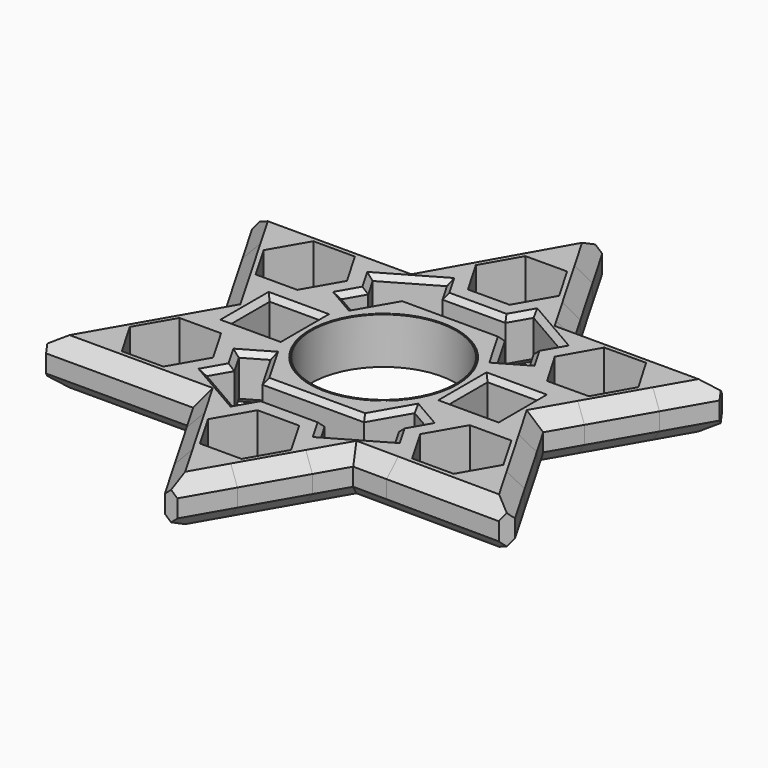
from build123d import *

# Parameters (mm, degrees)
F0_W     = 2.54
F0_H     = 8.7372876405
F0_H_2   = 8.9837514889
F1_DEPTH = 6.9977
F0_R     = 11.0653677003
F0_R_2   = 10.9474
F2_R     = 11.176
F3_DEPTH = 6.9977
F4_SIZE  = 2.159
F5_W     = 7.62
F5_H     = 7.62
F6_DEPTH = 25.4
F7_SIZE  = 0.762


with BuildPart() as f1:
    # F0 (on Top) → F1 (new body)
    with BuildSketch(Plane.XY):
        Polygon((12.5002051005, 12.7937514889), (14.280010725, 9.7110377198), (15.550010725, 7.5113331942), (17.2662315727, 4.5387514889), (20.7270452561, 4.5387514889), (23.2670452561, 4.5387514889), (26.798284517, 4.5387514889), (31.5643109892, 12.7937514889), (26.798284517, 21.0487514889), (17.2662315727, 21.0487514889), (15.5094151394, 18.0058561669), (14.1988195539, 15.7358380246), align=None)
        Polygon((25.2207365934, 7.3534421339), (18.9150512132, 7.3122933889), (15.7265726647, 12.7526027439), (18.8437794963, 18.2340608439), (25.1494648765, 18.2752095889), (28.3379434251, 12.8349002339), align=None, mode=Mode.SUBTRACT)
        Polygon((35.3419193782, -19.304), (31.5290982004, -12.7), (26.7630717283, -20.955), (17.231018784, -20.955), (34.3130483735, -21.0860568545), align=None)
        Polygon((4.7660264722, -33.655), (-4.7660264722, -33.655), (-0.9532052944, -40.259), (0.9532052944, -40.259), align=None)
        Polygon((-14.2130055479, -9.6723522628), (-15.4830055479, -7.4726477372), (-17.231018784, -4.445), (-20.7270452561, -4.445), (-23.2670452561, -4.445), (-26.7630717283, -4.445), (-31.5290982004, -12.7), (-26.7630717283, -20.955), (-17.231018784, -20.955), (-15.4830055479, -17.9273522628), (-14.2130055479, -15.7276477372), (-12.4649923118, -12.7), align=None)
        Polygon((-25.1531495269, -7.2408455632), (-18.847330966, -7.2371563061), (-15.6912266952, -12.6963107429), (-18.8409409854, -18.1591544368), (-25.1467595462, -18.1628436939), (-28.302863817, -12.7036892571), align=None, mode=Mode.SUBTRACT)
        with Locations((-21.9970452561, -0.0763561798)):
            Rectangle(F0_W, F0_H)
        Polygon((-35.2537508563, 19.1512876405), (-31.4409296786, 12.5472876405), (-29.0579164425, 16.6747876405), (-34.7771482091, 19.9767876405), align=None)
        Polygon((-29.0579164425, 16.6747876405), (-26.6749032064, 20.8022876405), (-34.3005455619, 20.8022876405), (-34.7771482091, 19.9767876405), align=None)
        Polygon((-14.2130055479, 15.7276477372), (-14.124837026, 15.5749353777), (-6.4258711864, 20.0199353777), (-7.6958711864, 22.2196399033), (-10.1507973178, 20.8022876405), (-15.394837026, 17.7746399033), align=None)
        Polygon((6.6462924911, 20.0962915574), (14.1988195539, 15.7358380246), (15.5094151394, 18.0058561669), (10.2389658396, 21.0487514889), (7.9568880766, 22.3663096997), align=None)
        with Locations((21.9970452561, 0.0468757445)):
            Rectangle(F0_W, F0_H_2)
        Polygon((15.4830055479, -17.9273522628), (14.2130055479, -15.7276477372), (6.5140397082, -20.1726477372), (7.7840397082, -22.3723522628), align=None)
        Polygon((-6.5140397082, -20.1726477372), (-14.2130055479, -15.7276477372), (-15.4830055479, -17.9273522628), (-7.7840397082, -22.3723522628), align=None)
        Polygon((-7.6958711864, 22.2196399033), (-6.4258711864, 20.0199353777), (-4.6778579503, 16.9922876405), (-1.27, 16.9922876405), (1.27, 16.9922876405), (4.854194994, 16.9922876405), (6.6462924911, 20.0962915574), (7.9568880766, 22.3663096997), (9.6202214662, 25.2472876405), (4.854194994, 33.5022876405), (-4.6778579503, 33.5022876405), (-9.4438844224, 25.2472876405), align=None)
        Polygon((6.3939514928, 25.2687924658), (3.2596837324, 19.7970718096), (-3.0460992385, 19.7755669843), (-6.217614449, 25.2257828151), (-3.0833466886, 30.6975034713), (3.2224362823, 30.7190082967), align=None, mode=Mode.SUBTRACT)
        Polygon((-4.7660264722, -17.145), (-6.5140397082, -20.1726477372), (-7.7840397082, -22.3723522628), (-9.5320529443, -25.4), (-4.7660264722, -33.655), (4.7660264722, -33.655), (9.5320529443, -25.4), (7.7840397082, -22.3723522628), (6.5140397082, -20.1726477372), (4.7660264722, -17.145), (1.27, -17.145), (-1.27, -17.145), align=None)
        Polygon((-6.3058196401, -25.4), (-3.15290982, -19.939), (3.15290982, -19.939), (6.3058196401, -25.4), (3.15290982, -30.861), (-3.15290982, -30.861), align=None, mode=Mode.SUBTRACT)
        Polygon((17.231018784, -4.445), (15.4830055479, -7.4726477372), (14.2130055479, -9.6723522628), (12.4649923118, -12.7), (14.2130055479, -15.7276477372), (15.4830055479, -17.9273522628), (17.231018784, -20.955), (26.7630717283, -20.955), (31.5290982004, -12.7), (26.7630717283, -4.445), (23.2670452561, -4.445), (20.7270452561, -4.445), align=None)
        Polygon((18.8463996297, -18.1623066071), (15.6912261579, -12.7026141527), (18.8418717843, -7.2403075456), (25.1476908826, -7.2376933929), (28.3028643543, -12.6973858473), (25.1522187279, -18.1596924544), align=None, mode=Mode.SUBTRACT)
        Polygon((-15.3507527651, 7.3962915574), (-14.0807527651, 9.595996083), (-12.3768237899, 12.5472876405), (-14.124837026, 15.5749353777), (-14.2130055479, 15.7276477372), (-15.394837026, 17.7746399033), (-17.1428502621, 20.8022876405), (-26.6749032064, 20.8022876405), (-29.0579164425, 16.6747876405), (-31.4409296786, 12.5472876405), (-26.6749032064, 4.2922876405), (-23.2670452561, 4.2922876405), (-20.7270452561, 4.2922876405), (-17.1428502621, 4.2922876405), align=None)
        Polygon((-18.7543705969, 18.0073656951), (-15.6030573636, 12.5454442165), (-18.7575635009, 7.0853661618), (-25.0633828715, 7.0872095858), (-28.2146961049, 12.5491310644), (-25.0601899676, 18.0092091191), align=None, mode=Mode.SUBTRACT)
        Polygon((-10.3635226281, -7.4498522628), (-11.6335226281, -5.2501477372), (-15.4830055479, -7.4726477372), (-14.2130055479, -9.6723522628), align=None)
        Polygon((15.4830055479, -7.4726477372), (11.6335226281, -5.2501477372), (10.3635226281, -7.4498522628), (14.2130055479, -9.6723522628), align=None)
        Polygon((14.280010725, 9.7110377198), (10.3635226281, 7.4498522628), (11.6335226281, 5.2501477372), (15.550010725, 7.5113331942), align=None)
        Polygon((-11.6335226281, 5.2501477372), (-10.3635226281, 7.4498522628), (-14.0807527651, 9.595996083), (-15.3507527651, 7.3962915574), align=None)
        Polygon((-26.7630717283, -20.955), (-31.5290982004, -12.7), (-35.3419193782, -19.304), (-34.3887140837, -20.955), align=None)
        Polygon((-23.2670452561, -4.445), (-23.2670452561, 4.2922876405), (-26.6749032064, 4.2922876405), (-24.1967497817, 0), (-26.7630717283, -4.445), align=None)
        Polygon((-17.1428502621, 20.8022876405), (-15.394837026, 17.7746399033), (-10.1507973178, 20.8022876405), (-11.9631661187, 20.8022876405), align=None)
        Polygon((-10.1507973178, 20.8022876405), (-7.6958711864, 22.2196399033), (-9.4438844224, 25.2472876405), (-11.9631661187, 20.8022876405), align=None)
        Polygon((10.2389658396, 21.0487514889), (15.5094151394, 18.0058561669), (17.2662315727, 21.0487514889), (12.0442474435, 21.0487514889), align=None)
        Polygon((26.798284517, 4.5387514889), (23.2670452561, 4.5387514889), (23.2670452561, -4.445), (26.7630717283, -4.445), (24.1778351231, 0), align=None)
        Polygon((-7.7840397082, -22.3723522628), (-15.4830055479, -17.9273522628), (-17.231018784, -20.955), (-12.0983748909, -20.955), (-9.5320529443, -25.4), align=None)
        Polygon((17.231018784, -20.955), (15.4830055479, -17.9273522628), (7.7840397082, -22.3723522628), (9.5320529443, -25.4), (12.1210099324, -20.9157949581), align=None)
        Polygon((-14.6646968374, 0), (-11.6335226281, 5.2501477372), (-15.3507527651, 7.3962915574), (-17.1428502621, 4.2922876405), (-20.7270452561, 4.2922876405), (-20.7270452561, -4.445), (-17.231018784, -4.445), (-15.4830055479, -7.4726477372), (-11.6335226281, -5.2501477372), align=None)
        Polygon((15.550010725, 7.5113331942), (11.6335226281, 5.2501477372), (14.6646968374, 0), (11.6335226281, -5.2501477372), (15.4830055479, -7.4726477372), (17.231018784, -4.445), (20.7270452561, -4.445), (20.7270452561, 4.5387514889), (17.2662315727, 4.5387514889), align=None)
        Polygon((-1.0222856092, 40.1062876405), (-9.4438844224, 25.2472876405), (-4.6778579503, 33.5022876405), (4.854194994, 33.5022876405), (1.0413738163, 40.1062876405), align=None)
        Polygon((7.9568880766, 22.3663096997), (10.2389658396, 21.0487514889), (12.0442474435, 21.0487514889), (12.0280142558, 21.0768681948), (9.6202214662, 25.2472876405), align=None)
        Polygon((34.4239268725, 21.0487514889), (26.798284517, 21.0487514889), (31.5643109892, 12.7937514889), (35.3771321669, 19.3977514889), align=None)
    extrude(amount=F1_DEPTH)

    # F2 (on Top) → F3 (join)
    with BuildSketch(Plane.XY):
        Polygon((7.6989658396, 13.335), (-7.6989658396, 13.335), (-15.3979316793, 0), (-7.6989658396, -13.335), (7.6989658396, -13.335), (15.3979316793, 0), align=None)
        Circle(F2_R, mode=Mode.SUBTRACT)
    extrude(amount=F3_DEPTH)

    # F4 (call 1 of 12: OpenCascade refuses the feature's edges together)
    f4_edges = [f1.edges().sort_by_distance(p)[0] for p in [
        (-29.72525, 9.575644, 0),
        (-29.769335, -9.652, 0),
    ]]
    chamfer(f4_edges, length=F4_SIZE)

    # F4#2 (call 2 of 12)
    f4_2_edges = [f1.edges().sort_by_distance(p)[0] for p in [
        (-29.72525, 9.575644, 6.9977),
        (-29.769335, -9.652, 6.9977),
    ]]
    chamfer(f4_2_edges, length=F4_SIZE)

    # F4#3 (call 3 of 12)
    f4_3_edges = [f1.edges().sort_by_distance(p)[0] for p in [
        (-23.131856, 20.802288, 0),
        (-6.492726, 30.454288, 0),
    ]]
    chamfer(f4_3_edges, length=F4_SIZE)

    # F4#4 (call 4 of 12)
    f4_4_edges = [f1.edges().sort_by_distance(p)[0] for p in [
        (-23.131856, 20.802288, 6.9977),
        (-6.492726, 30.454288, 6.9977),
    ]]
    chamfer(f4_4_edges, length=F4_SIZE)

    # F4#5 (call 5 of 12)
    f4_5_edges = [f1.edges().sort_by_distance(p)[0] for p in [
        (31.052496, -11.8745, 0),
        (29.777484, 9.698876, 0),
        (25.470453, -2.2225, 0),
    ]]
    chamfer(f4_5_edges, length=F4_SIZE)

    # F4#6 (call 6 of 12)
    f4_6_edges = [f1.edges().sort_by_distance(p)[0] for p in [
        (31.052496, -11.8745, 6.9977),
        (29.777484, 9.698876, 6.9977),
        (25.470453, -2.2225, 6.9977),
    ]]
    chamfer(f4_6_edges, length=F4_SIZE)

    # F4#7 (call 7 of 12)
    f4_7_edges = [f1.edges().sort_by_distance(p)[0] for p in [
        (23.234087, 21.048751, 0),
        (6.542811, 30.57752, 0),
    ]]
    chamfer(f4_7_edges, length=F4_SIZE)

    # F4#8 (call 8 of 12)
    f4_8_edges = [f1.edges().sort_by_distance(p)[0] for p in [
        (23.234087, 21.048751, 6.9977),
        (6.542811, 30.57752, 6.9977),
    ]]
    chamfer(f4_8_edges, length=F4_SIZE)

    # F4#9 (call 9 of 12)
    f4_9_edges = [f1.edges().sort_by_distance(p)[0] for p in [
        (23.217029, -21.000926, 0),
        (6.537108, -30.587397, 0),
    ]]
    chamfer(f4_9_edges, length=F4_SIZE)

    # F4#10 (call 10 of 12)
    f4_10_edges = [f1.edges().sort_by_distance(p)[0] for p in [
        (6.537108, -30.587397, 6.9977),
        (23.217029, -21.000926, 6.9977),
    ]]
    chamfer(f4_10_edges, length=F4_SIZE)

    # F4#11 (call 11 of 12)
    f4_11_edges = [f1.edges().sort_by_distance(p)[0] for p in [
        (-23.243544, -20.955, 0),
        (-6.52579, -30.607, 0),
    ]]
    chamfer(f4_11_edges, length=F4_SIZE)

    # F4#12 (call 12 of 12)
    f4_12_edges = [f1.edges().sort_by_distance(p)[0] for p in [
        (-23.243544, -20.955, 6.9977),
        (-6.52579, -30.607, 6.9977),
    ]]
    chamfer(f4_12_edges, length=F4_SIZE)

    # F5 (on face) → F6 (cut)
    with BuildSketch(Plane.XY.offset(6.9977)):
        with Locations((16.51, 0)):
            Rectangle(F5_W, F5_H)
        with Locations((-16.51, 0)):
            Rectangle(F5_W, F5_H)
    extrude(amount=-F6_DEPTH, mode=Mode.SUBTRACT)

    # F7
    f7_edges = [f1.edges().sort_by_distance(p)[0] for p in [
        (-10.275354, 17.797435, 0),
        (-10.275354, 17.797435, 6.9977),
        (10.422556, 17.916065, 6.9977),
        (10.422556, 17.916065, 0),
        (0.088169, 16.992288, 6.9977),
        (0.088169, 16.992288, 0),
        (-5.551865, 18.506112, 0),
        (-5.551865, 18.506112, 6.9977),
        (5.750244, 18.54429, 0),
        (5.750244, 18.54429, 6.9977),
        (13.349512, 14.264795, 6.9977),
        (13.390108, 11.252395, 6.9977),
        (12.59673, 8.739195, 6.9977),
        (9.306207, 10.551176, 6.9977),
        (0, 13.335, 6.9977),
        (-13.25083, 14.061112, 6.9977),
        (-13.228788, 11.071642, 6.9977),
        (-12.497101, 8.681674, 6.9977),
        (-9.306207, 10.551176, 6.9977),
        (-16.51, 3.81, 6.9977),
        (-20.32, 0, 6.9977),
        (-16.51, -3.81, 6.9977),
        (-12.7, 0, 6.9977),
        (16.51, 3.81, 6.9977),
        (20.32, 0, 6.9977),
        (16.51, -3.81, 6.9977),
        (12.7, 0, 6.9977),
        (12.563227, -8.719852, 6.9977),
        (9.306207, -10.551176, 6.9977),
        (0, -13.335, 6.9977),
        (-9.306207, -10.551176, 6.9977),
        (-12.563227, -8.719852, 6.9977),
        (-13.338999, -11.186176, 6.9977),
        (-13.338999, -14.213824, 6.9977),
        (-10.363523, -17.950148, 6.9977),
        (-5.640033, -18.658824, 6.9977),
        (0, -17.145, 6.9977),
        (5.640033, -18.658824, 6.9977),
        (10.363523, -17.950148, 6.9977),
        (13.338999, -14.213824, 6.9977),
        (13.338999, -11.186176, 6.9977),
        (-12.7, 0, 0),
        (10.363523, -17.950148, 0),
        (5.640033, -18.658824, 0),
        (-5.640033, -18.658824, 0),
        (-10.363523, -17.950148, 0),
        (13.390108, 11.252395, 0),
        (12.59673, 8.739195, 0),
        (13.349512, 14.264795, 0),
        (-9.306207, 10.551176, 0),
        (0, 13.335, 0),
        (-12.497101, 8.681674, 0),
        (-13.228788, 11.071642, 0),
        (-13.25083, 14.061112, 0),
        (16.51, -3.81, 0),
        (16.51, 3.81, 0),
        (12.7, 0, 0),
        (20.32, 0, 0),
        (-16.51, 3.81, 0),
        (-16.51, -3.81, 0),
        (-20.32, 0, 0),
        (0, -13.335, 0),
        (0, -17.145, 0),
        (-13.338999, -11.186176, 0),
        (-12.563227, -8.719852, 0),
        (12.563227, -8.719852, 0),
        (9.306207, -10.551176, 0),
        (-9.306207, -10.551176, 0),
        (13.338999, -11.186176, 0),
        (13.338999, -14.213824, 0),
    ]]
    chamfer(f7_edges, length=F7_SIZE)


with BuildPart() as f1b:
    # F0 (on Top) → F1, piece 2 (new body)
    with BuildSketch(Plane.XY):
        Circle(F0_R)
        Circle(F0_R_2, mode=Mode.SUBTRACT)
    extrude(amount=F1_DEPTH)


solid = Compound([f1.part, f1b.part])
